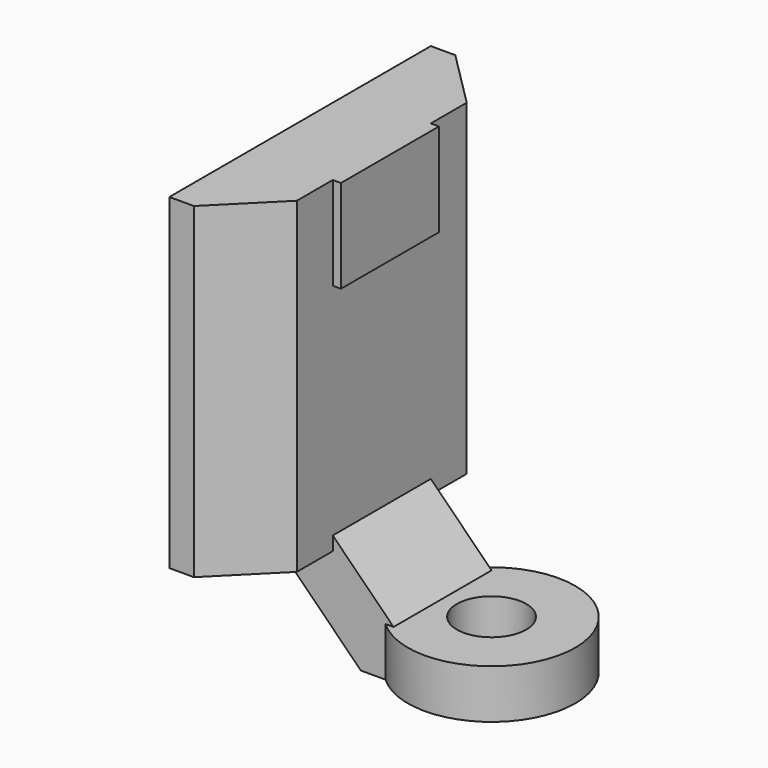
from build123d import *

# Parameters (mm, degrees)
F0_R     = 10.25
F0_R_2   = 4.25
F1_DEPTH = 6
F2_T     = -1
F4_DEPTH = 7.5
F6_DEPTH = 10
F7_SIZE  = 7


# Not quite as in the source:
# - a feature names something its author has since deleted; it is built from what else it names


with BuildPart() as f1:
    # F0 (on Top) → F1 (new body)
    with BuildSketch(Plane.XY):
        Circle(F0_R)
        Circle(F0_R_2, mode=Mode.SUBTRACT)
    extrude(amount=F1_DEPTH)

    # F2
    f2_openings = [f1.faces().sort_by_distance(p)[0] for p in [
        (-9.960086, 0, 0),
    ]]
    offset(amount=F2_T, openings=f2_openings)

    # F3 (on Front) → F4 (join, symmetric)
    with BuildSketch(Plane.XZ):
        Polygon((-23.44, 51.75), (-23.44, 13.44), (-10, 0), (-6, 0), (-6, 6), (-13.44, 13.44), (-13.44, 40.35), (-12.44, 40.35), (-12.44, 51.75), align=None)
    extrude(amount=F4_DEPTH, both=True)

    # F5 (on face) → F6 (join, through all)
    with BuildSketch(Plane(origin=(-23.44, 0, 0), x_dir=(0, -1, 0), z_dir=(-1, 0, 0))):
        with BuildLine():
            Line((20, 11.75), (20, 51.75))
            Line((20, 51.75), (7.5, 51.75))
            Line((7.5, 51.75), (7.5, 49.2070902501))
            ThreePointArc((7.5, 49.2070902501), (15.8666316526, 42.2022724802), (19, 31.75))
            ThreePointArc((19, 31.75), (15.8666316526, 21.2977275198), (7.5, 14.2929097499))
            Line((7.5, 14.2929097499), (7.5, 13.44))
            Line((7.5, 13.44), (5.0738446961, 13.44))
            ThreePointArc((5.0738446961, 13.44), (0, 12.75), (-5.0738446961, 13.44))
            Line((-5.0738446961, 13.44), (-7.5, 13.44))
            Line((-7.5, 13.44), (-7.5, 14.2929097499))
            ThreePointArc((-7.5, 14.2929097499), (-19, 31.75), (-7.5, 49.2070902501))
            Line((-7.5, 49.2070902501), (-7.5, 51.75))
            Line((-7.5, 51.75), (-20, 51.75))
            Line((-20, 51.75), (-20, 11.75))
            Line((-20, 11.75), (20, 11.75))
        make_face()
        with BuildLine():
            ThreePointArc((19, 31.75), (15.8666316526, 42.2022724802), (7.5, 49.2070902501))
            Line((7.5, 49.2070902501), (7.5, 14.2929097499))
            ThreePointArc((7.5, 14.2929097499), (15.8666316526, 21.2977275198), (19, 31.75))
        make_face()
        with BuildLine():
            Line((-7.5, 14.2929097499), (-7.5, 49.2070902501))
            ThreePointArc((-7.5, 49.2070902501), (-19, 31.75), (-7.5, 14.2929097499))
        make_face()
    extrude(amount=-F6_DEPTH)

    # F7
    f7_edges = [f1.edges().sort_by_distance(p)[0] for p in [
        (-13.44, -20, 31.75),
        (-13.44, 20, 31.75),
    ]]
    chamfer(f7_edges, length=F7_SIZE)


solid = f1.part
